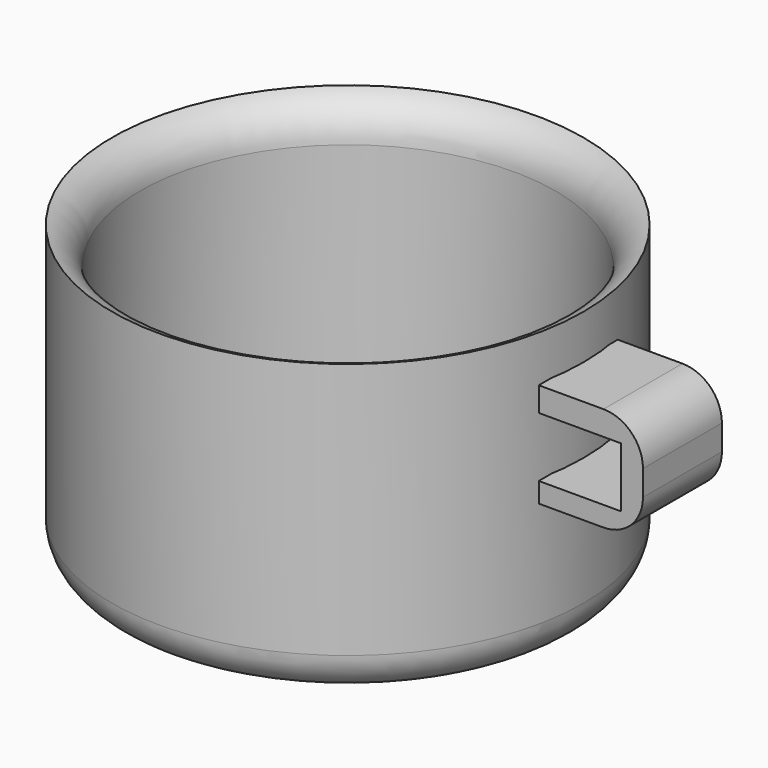
from build123d import *

# Parameters (mm, degrees)
F0_R     = 30.3392677901
F0_R_2   = 26.724855518
F1_DEPTH = 38.1
F2_R     = 26.7339886214
F3_DEPTH = 6.35
F5_DEPTH = 12.7
F8_R     = 5.08


# Not quite as in the source:
# - a fillet or chamfer that OpenCascade refuses, or shapes differently, is made with other operations: its cross-section is extruded or revolved along the edge and cut away or added


with BuildPart() as f1:
    # F0 (on Top) → F1 (new body)
    with BuildSketch(Plane.XY):
        Circle(F0_R)
        Circle(F0_R_2, mode=Mode.SUBTRACT)
    extrude(amount=F1_DEPTH)

    # F2 (on Top) → F3 (join)
    with BuildSketch(Plane.XY):
        Circle(F2_R)
    extrude(amount=F3_DEPTH)

    # F7: fillet of radius 5.08 on 2 edges, made by hand

    # F7_s1 → F7_t2 (revolve, cut)
    with BuildSketch(Plane.XZ):
        with BuildLine():
            ThreePointArc((30.3392677901, 38.1), (27.7273816887, 36.2659561382), (26.724855518, 33.2360044601))
            Line((26.724855518, 33.2360044601), (26.724855518, 38.1))
            Line((26.724855518, 38.1), (30.3392677901, 38.1))
        make_face()
    revolve(axis=Axis((0, 0, 38.1), (0, 0, 1)), mode=Mode.SUBTRACT)

    # F7_s3 → F7_t4 (revolve, cut)
    with BuildSketch(Plane.XZ):
        with BuildLine():
            ThreePointArc((30.3392677901, 5.08), (28.8513702385, 1.4878975516), (25.2592677901, 0))
            Line((25.2592677901, 0), (30.3392677901, 0))
            Line((30.3392677901, 0), (30.3392677901, 5.08))
        make_face()
    revolve(axis=Axis((0, 0, 0), (0, 0, 1)), mode=Mode.SUBTRACT)


with BuildPart() as f5:
    # F4 (on Front) → F5 (new body)
    with BuildSketch(Plane.XZ):
        Polygon((47.0647066832, 32.3748141527), (33.6583964527, 32.3748141527), (33.6583964527, 29.2371641845), (44.2123003304, 29.2371641845), (44.2123003304, 21.5356685221), (33.6583964527, 21.5356685221), (33.6583964527, 18.9685039222), (47.0647066832, 18.9685039222), align=None)
    extrude(amount=F5_DEPTH)


with BuildPart() as f5_1:
    # F6: moved
    add(f5.part.moved(Location((-3.70813, 5.99006, 0))))

    # F8
    f8_edges = [f5_1.edges().sort_by_distance(p)[0] for p in [
        (43.356577, -0.35994, 32.374814),
        (43.356577, -0.35994, 18.968504),
    ]]
    fillet(f8_edges, radius=F8_R)


solid = Compound([f1.part, f5_1.part])
